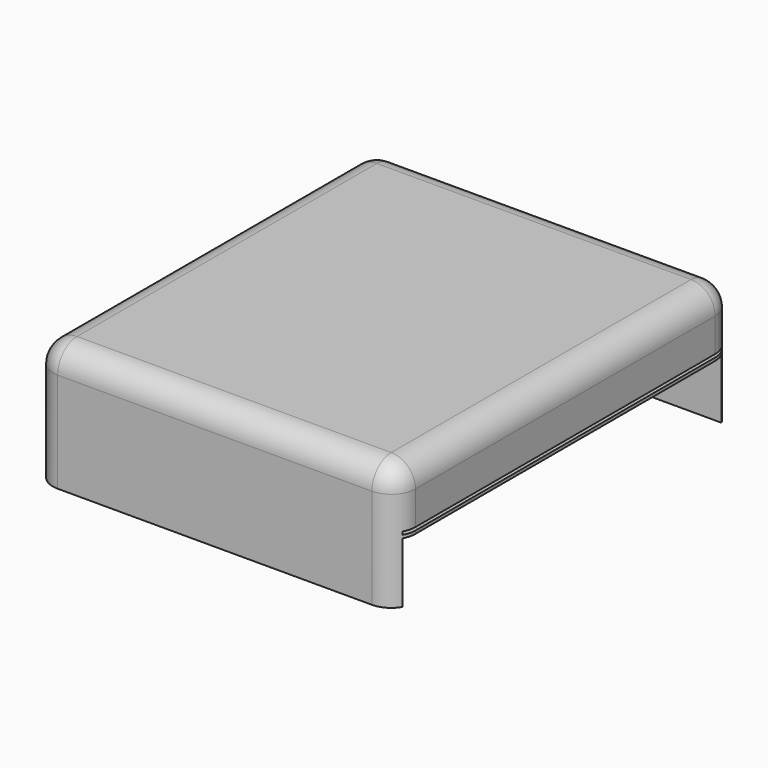
from build123d import *

# Parameters (mm, degrees)
F1_DEPTH     = 76.2
F2_W         = 83.8339800673
F2_H         = 0.635
F3_DEPTH     = 76.201
F4_W         = 71.12
F4_H         = 79.6544
F5_DEPTH     = 1.27
F6_R         = 5.08
F7_T1_DEPTH  = 33.7228350816
F7_S5_W      = 5.08
F7_S5_H      = 5.08
F7_T6_DEPTH  = 5.08
F8_T1_DEPTH  = 33.7228350816
F8_S5_W      = 5.08
F8_S5_H      = 5.08
F8_T6_DEPTH  = 5.08
F9_T1_DEPTH  = 33.7228350816
F9_S5_W      = 5.08
F9_S5_H      = 5.08
F9_T6_DEPTH  = 5.08
F10_T1_DEPTH = 33.7228350816
F10_S5_W     = 5.08
F10_S5_H     = 5.08
F10_T6_DEPTH = 5.08


# Not quite as in the source:
# - a fillet or chamfer that OpenCascade refuses, or shapes differently, is made with other operations: its cross-section is extruded or revolved along the edge and cut away or added


with BuildPart() as f1:
    # F0 (on Right) → F1 (new body)
    with BuildSketch(Plane.YZ):
        Polygon((0, 26.1028350816), (0, 0), (2.54, 0), (2.54, 12.7), (86.36, 12.7), (86.36, 0), (88.9, 0), (88.9, 26.1028350816), align=None)
    extrude(amount=-F1_DEPTH)

    # F2 (on face) → F3 (cut, through all)
    with BuildSketch(Plane.YZ):
        with Locations((44.4430099664, 13.6525)):
            Rectangle(F2_W, F2_H)
    extrude(amount=-F3_DEPTH, mode=Mode.SUBTRACT)

    # F4 (on face) → F5 (cut)
    with BuildSketch(Plane(origin=(0, 0, 12.7), x_dir=(1, 0, 0), z_dir=(0, 0, -1))):
        with Locations((-38.1, -44.45)):
            Rectangle(F4_W, F4_H)
    extrude(amount=-F5_DEPTH, mode=Mode.SUBTRACT)

    # F6
    f6_edges = [f1.edges().sort_by_distance(p)[0] for p in [
        (-38.1, 0, 26.102835),
        (0, 44.45, 26.102835),
        (-38.1, 88.9, 26.102835),
        (-76.2, 44.45, 26.102835),
    ]]
    fillet(f6_edges, radius=F6_R)

    # F7: fillet of radius 5.08 on 1 edges, made by hand

    # F7_s2 → F7_t1 (cut)
    with BuildSketch(Plane.XY.offset(-12.7)):
        with BuildLine():
            ThreePointArc((-5.08, 0), (-1.4878975516, 1.4878975516), (0, 5.08))
            Line((0, 5.08), (0, 0))
            Line((0, 0), (-5.08, 0))
        make_face()
    extrude(amount=F7_T1_DEPTH, mode=Mode.SUBTRACT)


with BuildPart() as f7_tool4:
    # F7_s5 → F7_t6 (new body)
    with BuildSketch(Plane.XZ.offset(-5.08)):
        with Locations((-2.54, 23.5628350816)):
            Rectangle(F7_S5_W, F7_S5_H)
    extrude(amount=F7_T6_DEPTH)

    # F7_s7 → F7_t8 (revolve, cut)
    with BuildSketch(Plane(origin=(-5.08, 5.08, 21.0228350816), x_dir=(-0.7071067812, 0, -0.7071067812), z_dir=(-0.7071067812, 0, 0.7071067812))):
        with BuildLine():
            ThreePointArc((0, -5.08), (5.08, 0), (0, 5.08))
            Line((0, 5.08), (0, -5.08))
        make_face()
    revolve(axis=Axis((-5.08, 5.08, 21.0228350816), (0, -1, 0)), mode=Mode.SUBTRACT)


with BuildPart() as f1_1:
    add(f1.part)

    # F7_t3: cut F7_tool4
    add(f7_tool4.part, mode=Mode.SUBTRACT)

    # F8: fillet of radius 5.08 on 1 edges, made by hand

    # F8_s2 → F8_t1 (cut)
    with BuildSketch(Plane.XY.offset(-12.7)):
        with BuildLine():
            ThreePointArc((0, 83.82), (-1.4878975516, 87.4121024484), (-5.08, 88.9))
            Line((-5.08, 88.9), (0, 88.9))
            Line((0, 88.9), (0, 83.82))
        make_face()
    extrude(amount=F8_T1_DEPTH, mode=Mode.SUBTRACT)


with BuildPart() as f8_tool4:
    # F8_s5 → F8_t6 (new body)
    with BuildSketch(Plane.YZ.offset(-5.08)):
        with Locations((86.36, 23.5628350816)):
            Rectangle(F8_S5_W, F8_S5_H)
    extrude(amount=F8_T6_DEPTH)

    # F8_s7 → F8_t8 (revolve, cut)
    with BuildSketch(Plane(origin=(-5.08, 83.82, 21.0228350816), x_dir=(0, -0.7071067812, -0.7071067812), z_dir=(0, -0.7071067812, 0.7071067812))):
        with BuildLine():
            ThreePointArc((0, -5.08), (5.08, 0), (0, 5.08))
            Line((0, 5.08), (0, -5.08))
        make_face()
    revolve(axis=Axis((-5.08, 83.82, 21.0228350816), (1, 0, 0)), mode=Mode.SUBTRACT)


with BuildPart() as f1_2:
    add(f1_1.part)

    # F8_t3: cut F8_tool4
    add(f8_tool4.part, mode=Mode.SUBTRACT)

    # F9: fillet of radius 5.08 on 1 edges, made by hand

    # F9_s2 → F9_t1 (cut)
    with BuildSketch(Plane.XY.offset(-12.7)):
        with BuildLine():
            ThreePointArc((-71.12, 0), (-74.7121024484, 1.4878975516), (-76.2, 5.08))
            Line((-76.2, 5.08), (-76.2, 0))
            Line((-76.2, 0), (-71.12, 0))
        make_face()
    extrude(amount=F9_T1_DEPTH, mode=Mode.SUBTRACT)


with BuildPart() as f9_tool4:
    # F9_s5 → F9_t6 (new body)
    with BuildSketch(Plane.XZ.offset(-5.08)):
        with Locations((-73.66, 23.5628350816)):
            Rectangle(F9_S5_W, F9_S5_H)
    extrude(amount=F9_T6_DEPTH)

    # F9_s7 → F9_t8 (revolve, cut)
    with BuildSketch(Plane(origin=(-71.12, 5.08, 21.0228350816), x_dir=(0.7071067812, 0, -0.7071067812), z_dir=(-0.7071067812, 0, -0.7071067812))):
        with BuildLine():
            ThreePointArc((0, -5.08), (5.08, 0), (0, 5.08))
            Line((0, 5.08), (0, -5.08))
        make_face()
    revolve(axis=Axis((-71.12, 5.08, 21.0228350816), (0, -1, 0)), mode=Mode.SUBTRACT)


with BuildPart() as f1_3:
    add(f1_2.part)

    # F9_t3: cut F9_tool4
    add(f9_tool4.part, mode=Mode.SUBTRACT)

    # F10: fillet of radius 5.08 on 1 edges, made by hand

    # F10_s2 → F10_t1 (cut)
    with BuildSketch(Plane.XY.offset(-12.7)):
        with BuildLine():
            ThreePointArc((-76.2, 83.82), (-74.7121024484, 87.4121024484), (-71.12, 88.9))
            Line((-71.12, 88.9), (-76.2, 88.9))
            Line((-76.2, 88.9), (-76.2, 83.82))
        make_face()
    extrude(amount=F10_T1_DEPTH, mode=Mode.SUBTRACT)


with BuildPart() as f10_tool4:
    # F10_s5 → F10_t6 (new body)
    with BuildSketch(Plane.YZ.offset(-71.12)):
        with Locations((86.36, 23.5628350816)):
            Rectangle(F10_S5_W, F10_S5_H)
    extrude(amount=-F10_T6_DEPTH)

    # F10_s7 → F10_t8 (revolve, cut)
    with BuildSketch(Plane(origin=(-71.12, 83.82, 21.0228350816), x_dir=(0, -0.7071067812, -0.7071067812), z_dir=(0, 0.7071067812, -0.7071067812))):
        with BuildLine():
            ThreePointArc((0, -5.08), (5.08, 0), (0, 5.08))
            Line((0, 5.08), (0, -5.08))
        make_face()
    revolve(axis=Axis((-71.12, 83.82, 21.0228350816), (-1, 0, 0)), mode=Mode.SUBTRACT)


with BuildPart() as f1_4:
    add(f1_3.part)

    # F10_t3: cut F10_tool4
    add(f10_tool4.part, mode=Mode.SUBTRACT)


solid = f1_4.part
